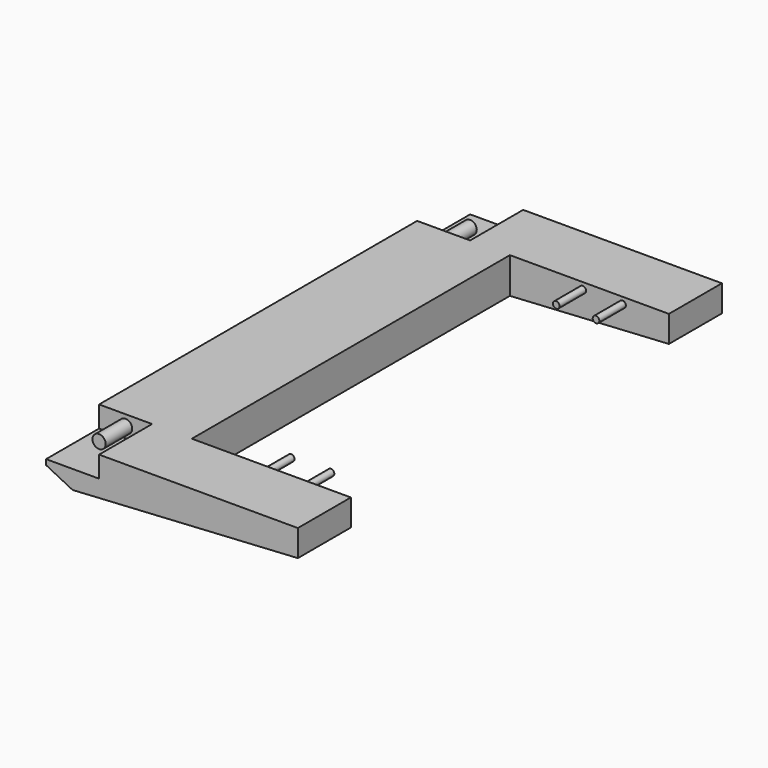
from build123d import *

# Parameters (mm, degrees)
F1_DEPTH = 50.8
F3_DEPTH = 7.621
F4_W     = 10.16
F4_H     = 4.064
F5_DEPTH = 12.7
F6_R     = 1.27
F7_DEPTH = 6.35
F8_R     = 0.635
F9_DEPTH = 6.35


# Not quite as in the source:
# - a pattern or mirror of a feature is missing from the dataset's text; its kind, count and spacing are read off the source's solid


with BuildPart() as f1:
    # F0 (on Front) → F1 (new body, symmetric)
    with BuildSketch(Plane.XZ):
        Polygon((-2.54, -4.9092677324), (-2.54, 0.1707322676), (-50.8, 0.1707322676), (-50.8, -4.9092677324), (-45.72, -7.4492677324), align=None)
    extrude(amount=F1_DEPTH, both=True)

    # F2 (on face) → F3 (cut, through all)
    with BuildSketch(Plane.XY.offset(0.1707322676)):
        Polygon((-2.54, 0), (-2.54, 38.1), (-33.02, 38.1), (-33.02, 0), (-33.02, -38.1), (-2.54, -38.1), align=None)
    extrude(amount=-F3_DEPTH, mode=Mode.SUBTRACT)

    # F4 (on face) → F5 (cut)
    with BuildSketch(Plane.XZ.offset(50.8)):
        with Locations((-45.72, -1.8612677324)):
            Rectangle(F4_W, F4_H)
    f5 = extrude(amount=-F5_DEPTH, mode=Mode.SUBTRACT)

    # F5_copies: F5 across plane
    add(f5.mirror(Plane.ZX), mode=Mode.SUBTRACT)

    # F6 (on face) → F7 (join)
    with BuildSketch(Plane.XZ.offset(38.1)):
        with Locations((-45.72, -1.8612677324)):
            Circle(F6_R)
    f7 = extrude(amount=F7_DEPTH)

    # F7_copies: F7 across plane
    add(f7.mirror(Plane.ZX))

    # F8 (on face) → F9 (join)
    with BuildSketch(Plane.XZ.offset(-38.1)):
        with Locations((-19.05, -1.0992677324)):
            Circle(F8_R)
        with Locations((-11.43, -1.0992677324)):
            Circle(F8_R)
    f9 = extrude(amount=F9_DEPTH)

    # F9_copies: F9 across plane
    add(f9.mirror(Plane(origin=(0, 0, 0), x_dir=(0, 0, -1), z_dir=(0, -1, 0))))


solid = f1.part
